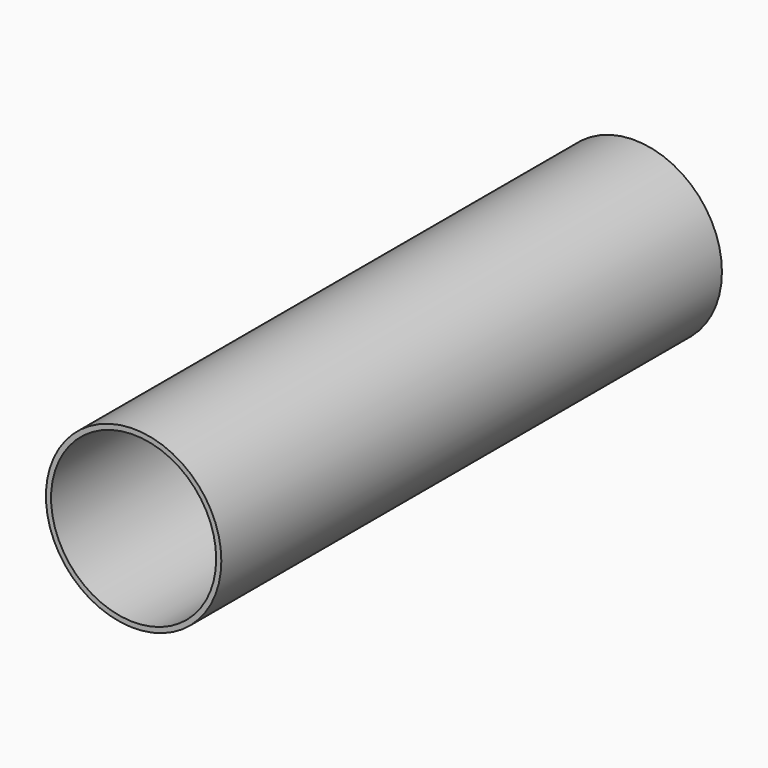
from build123d import *

# Parameters (mm, degrees)
F0_R     = 43.2566873222
F1_DEPTH = 308.61
F3_T     = -2.54


# Not quite as in the source:
# - the program builds the solid bodies; features that only make, move or delete a surface that nothing else refers to are left out


with BuildPart() as f1:
    # F0 (on Front) → F1 (new body)
    with BuildSketch(Plane.XZ):
        with Locations((-215.854883194, -11.3255027682)):
            Circle(F0_R)
    extrude(amount=-F1_DEPTH)

    # F3
    f3_openings = [f1.faces().sort_by_distance(p)[0] for p in [
        (-215.854883, 0, -11.325503),
    ]]
    offset(amount=F3_T, openings=f3_openings)


solid = f1.part
